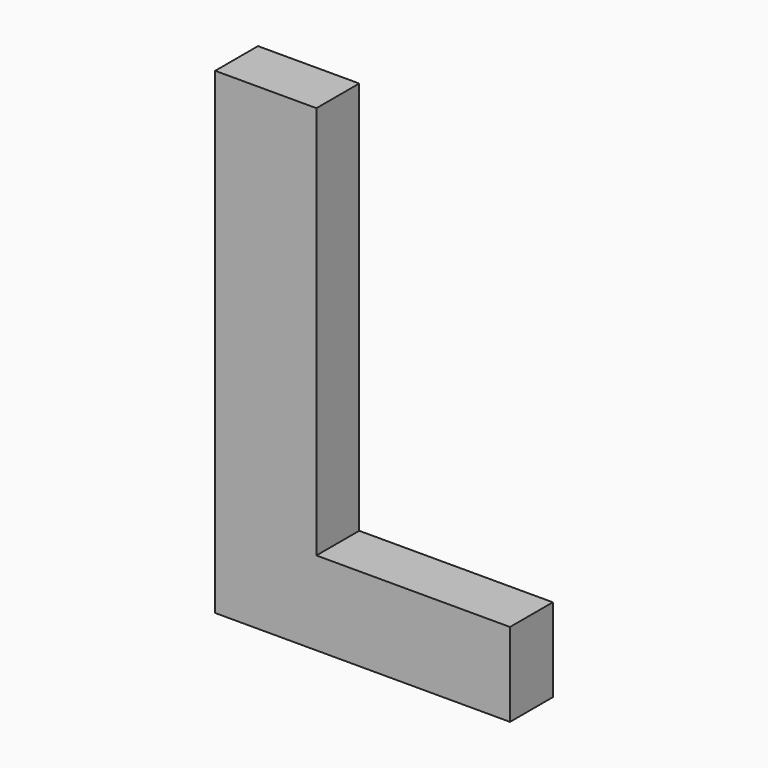
from build123d import *

# Parameters (mm, degrees)
F0_TEXT_SIZE = 62.5
F1_DEPTH     = 5


# Not quite as in the source:
# - Text() gives the source's letters only with a copy of the font that has no kerning and outlines rounded to 1/6400 em; it was checked with that copy


with BuildPart() as f1:
    # F0 (on Front) → F1 (new body)
    with BuildSketch(Plane.XZ):
        with Locations((-61.7471587042, 12.7840903935)):
            Text('L', F0_TEXT_SIZE, font='Open Sans', font_style=FontStyle.BOLD, text_align=(TextAlign.LEFT, TextAlign.BOTTOM))
    extrude(amount=F1_DEPTH)


solid = f1.part
